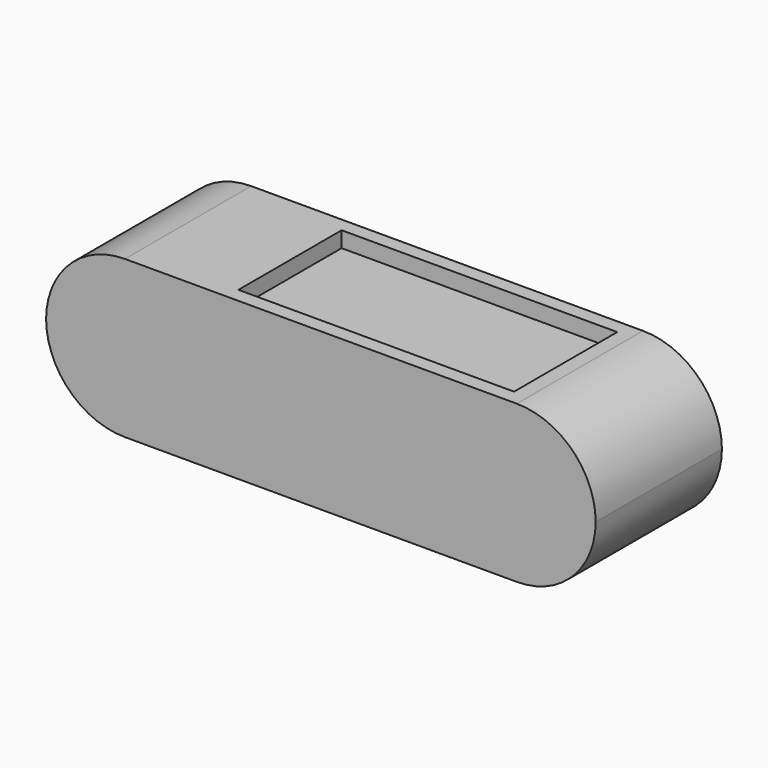
from build123d import *

# Parameters (mm, degrees)
F0_W        = 176.9779659808
F0_H        = 50.5181439221
F1_DEPTH    = 50.8
F2_T1_DEPTH = 177.8
F3_W        = 88.7552052736
F3_H        = 41.5458488278
F4_DEPTH    = 5.08


# Not quite as in the source:
# - a fillet or chamfer that OpenCascade refuses, or shapes differently, is made with other operations: its cross-section is extruded or revolved along the edge and cut away or added


with BuildPart() as f1:
    # F0 (on Front) → F1 (new body)
    with BuildSketch(Plane.XZ):
        with Locations((30.3119476885, -8.4089655429)):
            Rectangle(F0_W, F0_H)
    extrude(amount=F1_DEPTH)

    # F2: fillet of radius 25.4 on 4 edges, made by hand

    # F2_s2 → F2_t1 (cut)
    with BuildSketch(Plane.XZ.offset(-63.5)):
        with BuildLine():
            ThreePointArc((-32.7770353019, 16.8501064181), (-50.7375475441, 9.4106186603), (-58.1770353019, -8.5498935819))
            Line((-58.1770353019, -8.5498935819), (-58.1770353019, 16.8501064181))
            Line((-58.1770353019, 16.8501064181), (-32.7770353019, 16.8501064181))
        make_face()
        with BuildLine():
            ThreePointArc((-58.1770353019, -8.268037504), (-50.7375475441, -26.2285497461), (-32.7770353019, -33.668037504))
            Line((-32.7770353019, -33.668037504), (-58.1770353019, -33.668037504))
            Line((-58.1770353019, -33.668037504), (-58.1770353019, -8.268037504))
        make_face()
        with BuildLine():
            ThreePointArc((93.4009306788, 16.8501064181), (111.361442921, 9.4106186603), (118.8009306788, -8.5498935819))
            Line((118.8009306788, -8.5498935819), (118.8009306788, 16.8501064181))
            Line((118.8009306788, 16.8501064181), (93.4009306788, 16.8501064181))
        make_face()
        with BuildLine():
            ThreePointArc((93.4009306788, -33.668037504), (111.361442921, -26.2285497461), (118.8009306788, -8.268037504))
            Line((118.8009306788, -8.268037504), (118.8009306788, -33.668037504))
            Line((118.8009306788, -33.668037504), (93.4009306788, -33.668037504))
        make_face()
    extrude(amount=F2_T1_DEPTH, mode=Mode.SUBTRACT)

    # F3 (on face) → F4 (cut)
    with BuildSketch(Plane.XY.offset(16.8501064181)):
        with Locations((44.3776026368, -25.3384022508)):
            Rectangle(F3_W, F3_H)
    extrude(amount=-F4_DEPTH, mode=Mode.SUBTRACT)


solid = f1.part
